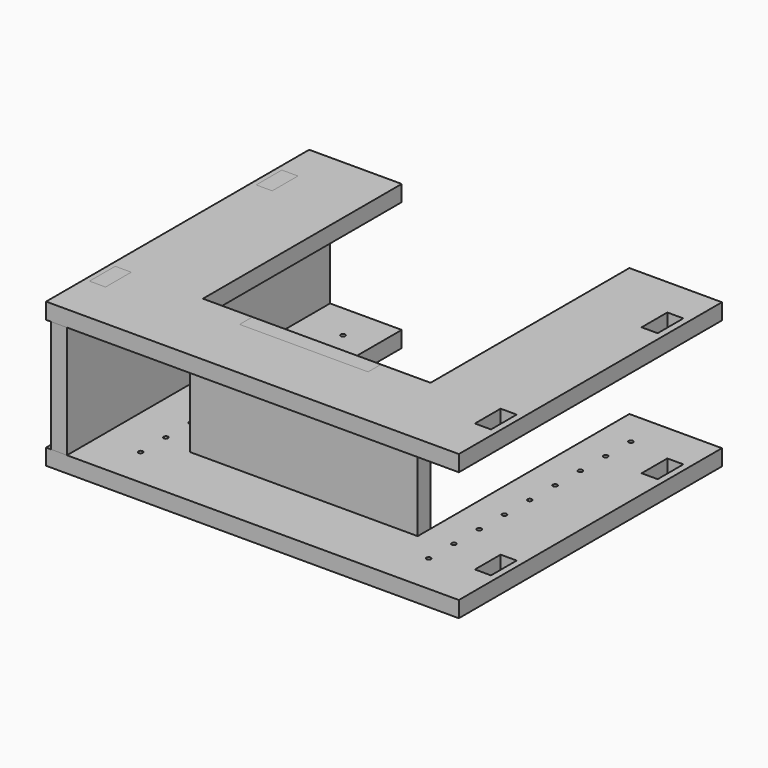
from build123d import *

# Parameters (mm, degrees)
F1_R      = 1.75
F1_W      = 12.7
F1_H      = 25.4
F2_DEPTH  = 12.7
F3_W      = 12.7
F3_H      = 139.35
F3_H_2    = 38.1
F3_H_3    = 25.4
F3_H_4    = 31.75
F4_DEPTH  = 88.9
F5_DEPTH  = 12.7
F6_W      = 12.7
F6_H      = 25.4
F6_H_2    = 139.35
F7_DEPTH  = 12.7
F9_W      = 101.6
F9_H      = 12.7
F10_DEPTH = 12.7


# Not quite as in the source:
# - a feature of the source that left no trace in its solid (it failed there, or was rolled back) is left out
# - a pattern or mirror of a feature is missing from the dataset's text; its kind, count and spacing are read off the source's solid


with BuildPart() as f2:
    # F1 (on Top) → F2 (new body)
    with BuildSketch(Plane.XY):
        Polygon((-128.2246859372, 152.7786509395), (-201.4082543561, 152.7786509395), (-201.4082543561, -107.2213490605), (124.9588824817, -107.2213490605), (124.9588824817, 152.7786509395), (51.7753140628, 152.7786509395), (51.7753140628, -43.7213490605), (12.5753140628, -43.7213490605), (12.5753140628, -56.4213490605), (-89.0246859372, -56.4213490605), (-89.0246859372, -43.7213490605), (-128.2246859372, -43.7213490605), align=None)
        with Locations((-152.0671993494, -75.4713490605)):
            Circle(F1_R, mode=Mode.SUBTRACT)
        with Locations((-191.2300288677, -56.4213490605)):
            Rectangle(F1_W, F1_H, mode=Mode.SUBTRACT)
        with Locations((-152.0671993494, -50.4713490605)):
            Circle(F1_R, mode=Mode.SUBTRACT)
        with Locations((-152.0671993494, -25.4713490605)):
            Circle(F1_R, mode=Mode.SUBTRACT)
        with Locations((-152.0671993494, -0.4713490605)):
            Circle(F1_R, mode=Mode.SUBTRACT)
        with Locations((75.6178274751, -75.4713490605)):
            Circle(F1_R, mode=Mode.SUBTRACT)
        with Locations((75.6178274751, -50.4713490605)):
            Circle(F1_R, mode=Mode.SUBTRACT)
        with Locations((113.5288824817, -56.4213490605)):
            Rectangle(F1_W, F1_H, mode=Mode.SUBTRACT)
        with Locations((75.6178274751, -25.4713490605)):
            Circle(F1_R, mode=Mode.SUBTRACT)
        with Locations((75.6178274751, -0.4713490605)):
            Circle(F1_R, mode=Mode.SUBTRACT)
        with Locations((-152.0671993494, 24.5286509395)):
            Circle(F1_R, mode=Mode.SUBTRACT)
        with Locations((-152.0671993494, 49.5286509395)):
            Circle(F1_R, mode=Mode.SUBTRACT)
        with Locations((-152.0671993494, 74.5286509395)):
            Circle(F1_R, mode=Mode.SUBTRACT)
        with Locations((-191.2300288677, 108.3286509395)):
            Rectangle(F1_W, F1_H, mode=Mode.SUBTRACT)
        with Locations((-152.0671993494, 99.5286509395)):
            Circle(F1_R, mode=Mode.SUBTRACT)
        with Locations((-152.0671993494, 124.5286509395)):
            Circle(F1_R, mode=Mode.SUBTRACT)
        with Locations((75.6178274751, 24.5286509395)):
            Circle(F1_R, mode=Mode.SUBTRACT)
        with Locations((75.6178274751, 49.5286509395)):
            Circle(F1_R, mode=Mode.SUBTRACT)
        with Locations((75.6178274751, 74.5286509395)):
            Circle(F1_R, mode=Mode.SUBTRACT)
        with Locations((75.6178274751, 99.5286509395)):
            Circle(F1_R, mode=Mode.SUBTRACT)
        with Locations((113.5288824817, 108.3286509395)):
            Rectangle(F1_W, F1_H, mode=Mode.SUBTRACT)
        with Locations((75.6178274751, 124.5286509395)):
            Circle(F1_R, mode=Mode.SUBTRACT)
    extrude(amount=F2_DEPTH)


with BuildPart() as f4:
    # F3 (on face) → F4 (new body)
    with BuildSketch(Plane.XY.offset(12.7)):
        with Locations((-191.2300288677, 25.9536509395)):
            Rectangle(F3_W, F3_H)
        with Locations((-191.2300288677, -88.1713490605)):
            Rectangle(F3_W, F3_H_2)
        with Locations((-191.2300288677, 108.3286509395)):
            Rectangle(F3_W, F3_H_3)
        with Locations((-191.2300288677, 136.9036509395)):
            Rectangle(F3_W, F3_H_4)
        with Locations((-191.2300288677, -56.4213490605)):
            Rectangle(F3_W, F3_H_3)
    extrude(amount=F4_DEPTH)

    # F3 (on face) → F5 (join, through all)
    with BuildSketch(Plane.XY.offset(12.7)):
        with Locations((-191.2300288677, -56.4213490605)):
            Rectangle(F3_W, F3_H_3)
        with Locations((-191.2300288677, 108.3286509395)):
            Rectangle(F3_W, F3_H_3)
    f5 = extrude(amount=-F5_DEPTH)

    # F5_copies: F5 across plane
    add(f5.mirror(Plane.XY.offset(57.15)))


with BuildPart() as f7:
    # F6 (on face) → F7 (new body)
    with BuildSketch(Plane.XY.offset(101.6)):
        Polygon((-128.2246859372, 152.7786509395), (-201.4082543561, 152.7786509395), (-201.4082543561, -107.2213490605), (124.9588824817, -107.2213490605), (124.9588824817, 152.7786509395), (51.7753140628, 152.7786509395), (51.7753140628, -43.7213490605), (12.5753140628, -43.7213490605), (12.5753140628, -56.4213490605), (-89.0246859372, -56.4213490605), (-89.0246859372, -43.7213490605), (-128.2246859372, -43.7213490605), align=None)
        with Locations((113.5288824817, -56.4213490605)):
            Rectangle(F6_W, F6_H, mode=Mode.SUBTRACT)
        Polygon((-197.5800288677, -43.7213490605), (-197.5800288677, 95.6286509395), (-197.5800288677, 121.0286509395), (-184.8800288677, 121.0286509395), (-184.8800288677, 95.6286509395), (-184.8800288677, -43.7213490605), (-184.8800288677, -69.1213490605), (-197.5800288677, -69.1213490605), align=None, mode=Mode.SUBTRACT)
        with Locations((113.5288824817, 108.3286509395)):
            Rectangle(F6_W, F6_H, mode=Mode.SUBTRACT)
        with Locations((-191.2300288677, 25.9536509395)):
            Rectangle(F6_W, F6_H_2)
    extrude(amount=F7_DEPTH)


with BuildPart() as f10:
    # F9 (on face) → F10 (new body, through all)
    with BuildSketch(Plane(origin=(0, -56.4213490605, 0), x_dir=(-1, 0, 0), z_dir=(0, 1, 0))):
        Polygon((89.0246859372, 101.6), (-12.5753140628, 101.6), (-51.7753140628, 101.6), (-51.7753140628, 12.7), (-12.5753140628, 12.7), (-12.5753140628, 0), (89.0246859372, 0), (89.0246859372, 12.7), (128.2246859372, 12.7), (128.2246859372, 101.6), align=None)
        with Locations((38.2246859372, 107.95)):
            Rectangle(F9_W, F9_H)
    extrude(amount=F10_DEPTH)


solid = Compound([f2.part, f4.part, f7.part, f10.part])
